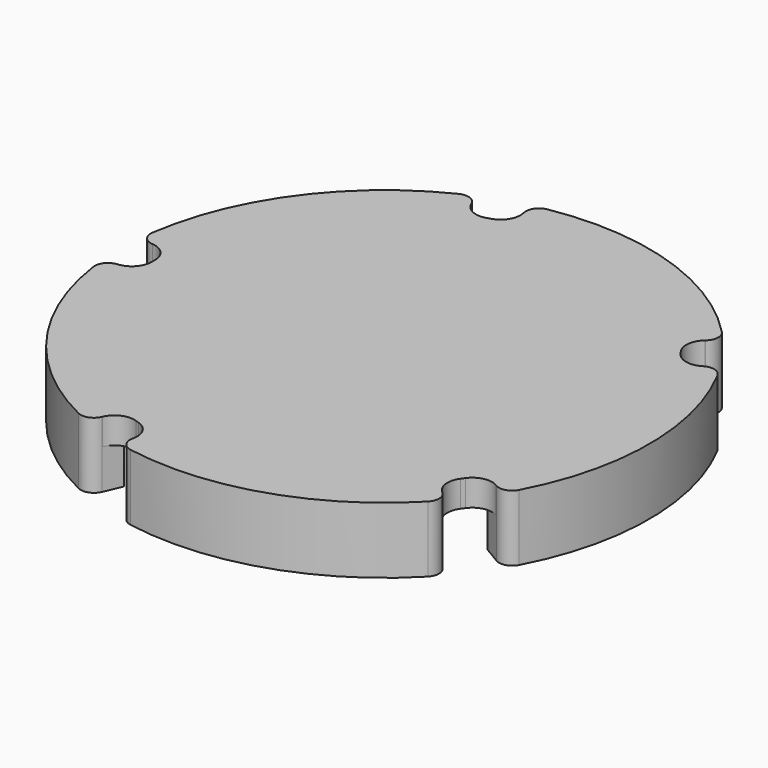
from build123d import *

# Parameters (mm, degrees)
F1_DEPTH      = 2
F2_DEPTH      = 2
F2_DEPTH_BACK = 3
F3_R          = 1.5
F4_R          = 1


with BuildPart() as f1:
    # F0 (on Top) → F1 (new body)
    with BuildSketch(Plane.XY):
        with BuildLine():
            ThreePointArc((15.0004277623, -9.0131663109), (16.8635329312, -4.6766715814), (17.5, 0))
            ThreePointArc((17.5, 0), (16.8635329312, 4.6766715814), (15.0004277623, 9.0131663109))
            ThreePointArc((15.0004277623, 9.0131663109), (14.1577974016, 10.2862419151), (13.2074176539, 11.4810330073))
            ThreePointArc((13.2074176539, 11.4810330073), (5.4077974016, 16.6434890352), (-3.936643451, 17.0514761337))
            ThreePointArc((-3.936643451, 17.0514761337), (-5.4077974016, 16.6434890352), (-6.8377947486, 16.1088349354))
            ThreePointArc((-6.8377947486, 16.1088349354), (-14.1577974016, 10.2862419151), (-17.4334072166, 1.5252254981))
            ThreePointArc((-17.4334072166, 1.5252254981), (-17.5, 0), (-17.4334072166, -1.5252254981))
            ThreePointArc((-17.4334072166, -1.5252254981), (-14.1577974016, -10.2862419151), (-6.8377947486, -16.1088349354))
            ThreePointArc((-6.8377947486, -16.1088349354), (-5.4077974016, -16.6434890352), (-3.936643451, -17.0514761337))
            ThreePointArc((-3.936643451, -17.0514761337), (5.4077974016, -16.6434890352), (13.2074176539, -11.4810330073))
            ThreePointArc((13.2074176539, -11.4810330073), (14.1577974016, -10.2862419151), (15.0004277623, -9.0131663109))
        make_face()
    extrude(amount=F1_DEPTH)

    # F0 (on Top) → F2 (join, two sides)
    with BuildSketch(Plane.XY) as f2_sk:
        with BuildLine():
            ThreePointArc((15.0004277623, 9.0131663109), (16.8635329312, 4.6766715814), (17.5, 0))
            ThreePointArc((17.5, 0), (16.8635329312, -4.6766715814), (15.0004277623, -9.0131663109))
            Line((15.0004277623, -9.0131663109), (17.143346014, -10.3007614982))
            ThreePointArc((17.143346014, -10.3007614982), (20, 0), (17.143346014, 10.3007614982))
            Line((17.143346014, 10.3007614982), (15.0004277623, 9.0131663109))
        make_face()
        with BuildLine():
            ThreePointArc((-3.936643451, 17.0514761337), (5.4077974016, 16.6434890352), (13.2074176539, 11.4810330073))
            Line((13.2074176539, 11.4810330073), (15.0941916045, 13.1211805798))
            ThreePointArc((15.0941916045, 13.1211805798), (6.1803398875, 19.0211303259), (-4.4990210869, 19.4874012957))
            Line((-4.4990210869, 19.4874012957), (-3.936643451, 17.0514761337))
        make_face()
        with BuildLine():
            ThreePointArc((-17.4334072166, 1.5252254981), (-14.1577974016, 10.2862419151), (-6.8377947486, 16.1088349354))
            Line((-6.8377947486, 16.1088349354), (-7.8146225698, 18.410097069))
            ThreePointArc((-7.8146225698, 18.410097069), (-16.1803398875, 11.7557050458), (-19.9238939618, 1.743114855))
            Line((-19.9238939618, 1.743114855), (-17.4334072166, 1.5252254981))
        make_face()
        with BuildLine():
            Line((-7.8146225698, -18.410097069), (-6.8377947486, -16.1088349354))
            ThreePointArc((-6.8377947486, -16.1088349354), (-14.1577974016, -10.2862419151), (-17.4334072166, -1.5252254981))
            Line((-17.4334072166, -1.5252254981), (-19.9238939618, -1.743114855))
            ThreePointArc((-19.9238939618, -1.743114855), (-16.1803398875, -11.7557050458), (-7.8146225698, -18.410097069))
        make_face()
        with BuildLine():
            Line((15.0941916045, -13.1211805798), (13.2074176539, -11.4810330073))
            ThreePointArc((13.2074176539, -11.4810330073), (5.4077974016, -16.6434890352), (-3.936643451, -17.0514761337))
            Line((-3.936643451, -17.0514761337), (-4.4990210869, -19.4874012957))
            ThreePointArc((-4.4990210869, -19.4874012957), (6.1803398875, -19.0211303259), (15.0941916045, -13.1211805798))
        make_face()
    extrude(amount=F2_DEPTH)
    extrude(f2_sk.sketch, amount=-F2_DEPTH_BACK)

    # F3
    f3_edges = [f1.edges().sort_by_distance(p)[0] for p in [
        (-17.433407, 1.525225, 1),
        (-17.433407, -1.525225, 1),
        (-3.936643, -17.051476, 1),
        (-6.837795, -16.108835, 1),
        (15.000428, -9.013166, 1),
        (13.207418, -11.481033, 1),
        (13.207418, 11.481033, 1),
        (15.000428, 9.013166, 1),
        (-6.837795, 16.108835, 1),
        (-3.936643, 17.051476, 1),
    ]]
    fillet(f3_edges, radius=F3_R)

    # F4
    f4_edges = [f1.edges().sort_by_distance(p)[0] for p in [
        (15.094192, -13.121181, -0.5),
        (17.143346, -10.300761, -0.5),
        (17.143346, 10.300761, -0.5),
        (15.094192, 13.121181, -0.5),
        (-4.499021, 19.487401, -0.5),
        (-7.814623, 18.410097, -0.5),
        (-19.923894, 1.743115, -0.5),
        (-19.923894, -1.743115, -0.5),
        (-4.499021, -19.487401, -0.5),
        (-7.814623, -18.410097, -0.5),
    ]]
    fillet(f4_edges, radius=F4_R)


solid = f1.part
